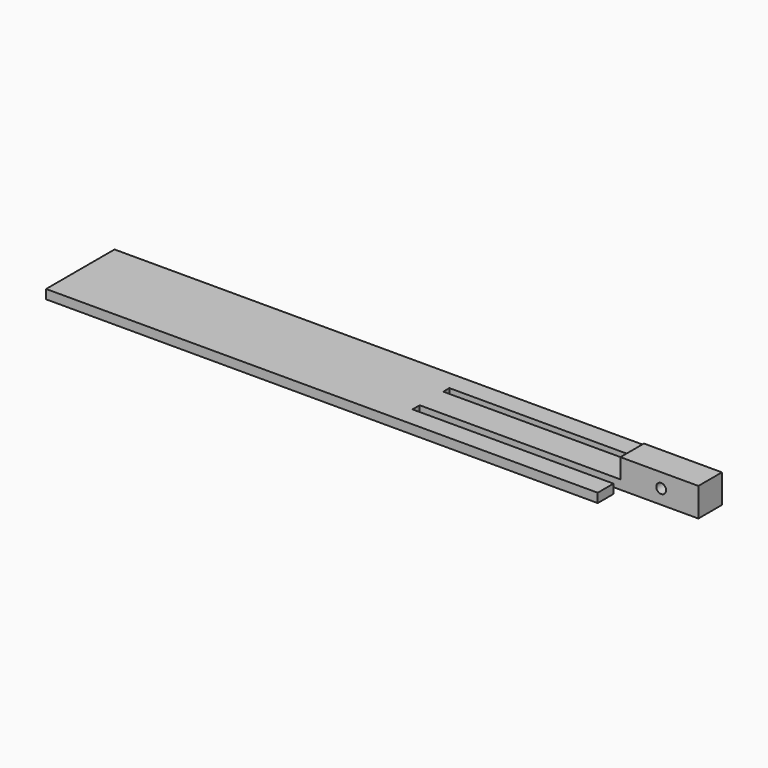
from build123d import *

# Parameters (mm, degrees)
F1_DEPTH = 2.8
F2_DEPTH = 23.8
F3_DEPTH = 23.89
F4_DEPTH = 42.8
F5_W     = 23.89
F5_H     = 9.0229478665
F6_DEPTH = 6
F7_R     = 1.5
F8_DEPTH = 9.0229478665
F9_DEPTH = 1.439


with BuildPart() as f1:
    # F0 (on Top) → F1 (new body)
    with BuildSketch(Plane.XY):
        Polygon((-75.0034600496, -12.3867541552), (75.0034600496, -12.3867541552), (75.0034600496, -6.3421353698), (-10.3727839887, -6.3421353698), (-10.3727839887, -3.5960208625), (75.0034600496, -3.5960208625), (75.0034600496, 5.426927004), (-10.3727839887, 5.426927004), (-10.3727839887, 7.7807395719), (75.0034600496, 7.7807395719), (75.0034600496, 12.3867541552), (-75.0034600496, 12.3867541552), align=None)
    extrude(amount=F1_DEPTH)

    # F2 (cut): a face of the model
    f2_faces = [f1.faces().sort_by_distance(p)[0] for p in [
        (75.0034600496, -9.3644447625, 1.4),
    ]]
    extrude(f2_faces, amount=-F2_DEPTH, mode=Mode.SUBTRACT)

    # F3 (cut): a face of the model
    f3_faces = [f1.faces().sort_by_distance(p)[0] for p in [
        (75.0034600496, 10.0837468635, 1.4),
    ]]
    extrude(f3_faces, amount=-F3_DEPTH, mode=Mode.SUBTRACT)

    # F4 (add): a face of the model
    f4_faces = [f1.faces().sort_by_distance(p)[0] for p in [
        (-75.0034600496, 0, 1.4),
    ]]
    extrude(f4_faces, amount=F4_DEPTH)

    # F5 (on face) → F6 (join)
    with BuildSketch(Plane.XY.offset(2.8)):
        with Locations((63.0584600496, 0.9154530708)):
            Rectangle(F5_W, F5_H)
    extrude(amount=F6_DEPTH)

    # F7 (on face) → F8 (cut, through all)
    with BuildSketch(Plane.XZ.offset(3.5960208625)):
        with Locations((63.6097043753, 4.4)):
            Circle(F7_R)
    extrude(amount=-F8_DEPTH, mode=Mode.SUBTRACT)

    # F9 (add): a face of the model
    f9_faces = [f1.faces().sort_by_distance(p)[0] for p in [
        (-33.345, 12.3867541552, 1.4),
    ]]
    extrude(f9_faces, amount=F9_DEPTH)


solid = f1.part
